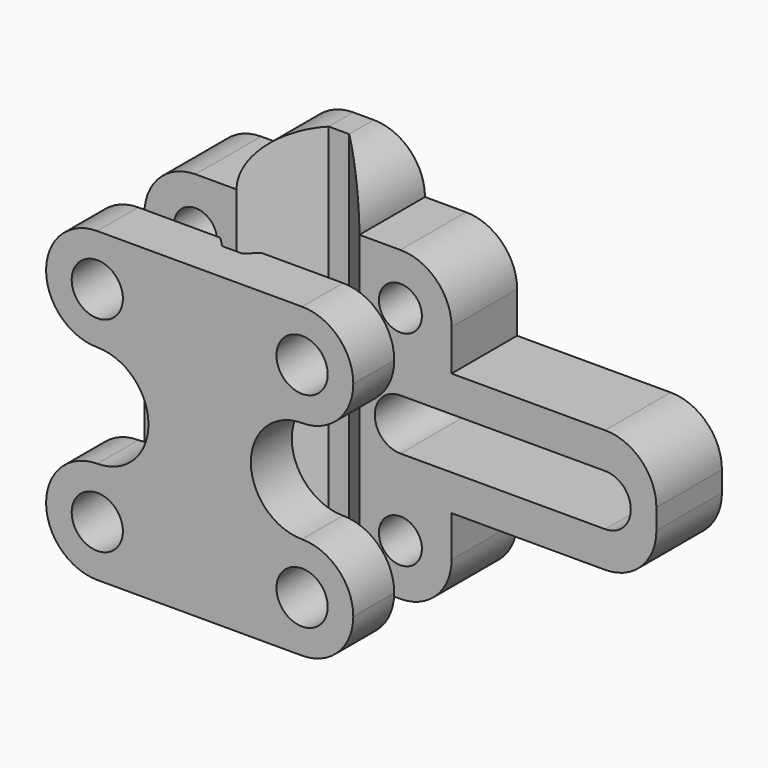
from build123d import *

# Parameters (mm, degrees)
F0_R      = 2.5
F1_DEPTH  = 8
F3_DEPTH  = 40
F4_D      = 4.2
F5_R      = 4.99999
F7_DEPTH  = 5
F8_D      = 5
F9_R      = 5
F11_DEPTH = 50
F13_R     = 4.99999


# Not quite as in the source:
# - a fillet or chamfer is up to 0.001 mm smaller than in the source, because OpenCascade refuses the exact size


with BuildPart() as f1:
    # F0 (on Front) → F1 (new body)
    with BuildSketch(Plane.XZ):
        Polygon((24, 0), (36, 0), (36, 5), (45, 5), (45, 14), (65, 14), (65, 26), (45, 26), (45, 35), (36, 35), (36, 40), (24, 40), (24, 35), (15, 35), (15, 26), (15, 14), (15, 5), (24, 5), align=None)
        with Locations((20, 20)):
            Circle(F0_R, mode=Mode.SUBTRACT)
        with BuildLine():
            ThreePointArc((40, 17.5), (37.5, 20), (40, 22.5))
            Line((40, 22.5), (60, 22.5))
            ThreePointArc((60, 22.5), (62.5, 20), (60, 17.5))
            Line((60, 17.5), (40, 17.5))
        make_face(mode=Mode.SUBTRACT)
    extrude(amount=F1_DEPTH)

    # F2 (on Top) → F3 (cut)
    with BuildSketch(Plane.XY):
        Polygon((29, -3), (24, -8), (36, -8), (31, -3), align=None)
    extrude(amount=F3_DEPTH, mode=Mode.SUBTRACT)

    # F4 (through all)
    with Locations(Plane(origin=(0, 0, 0), x_dir=(1, 0, 0), z_dir=(0, 1, 0))):
        with Locations((20, -30), (40, -30), (40, -10), (20, -10)):
            Hole(F4_D / 2)

    # F5 (radius 5 in the source; OpenCascade refuses exactly that, so slightly less here)
    f5_edges = [f1.edges().sort_by_distance(p)[0] for p in [
        (36, -4, 40),
        (24, -4, 40),
        (45, -4, 35),
        (15, -4, 35),
        (15, -4, 5),
        (36, -4, 0),
        (24, -4, 0),
        (45, -4, 5),
        (65, -4, 26),
        (65, -4, 14),
    ]]
    fillet(f5_edges, radius=F5_R)


with BuildPart() as f7:
    # F6 (on Front) → F7 (new body)
    with BuildSketch(Plane.XZ):
        with BuildLine():
            Line((45, 25), (45, 35))
            Line((45, 35), (15, 35))
            Line((15, 35), (15, 25))
            Line((15, 25), (20, 25))
            ThreePointArc((20, 25), (25, 20), (20, 15))
            Line((20, 15), (15, 15))
            Line((15, 15), (15, 5))
            Line((15, 5), (45, 5))
            Line((45, 5), (45, 15))
            Line((45, 15), (40, 15))
            ThreePointArc((40, 15), (35, 20), (40, 25))
            Line((40, 25), (45, 25))
        make_face()
    extrude(amount=F7_DEPTH)

    # F8 (through all)
    with Locations(Plane(origin=(0, 0, 0), x_dir=(1, 0, 0), z_dir=(0, 1, 0))):
        with Locations((40, -30), (20, -30), (20, -10), (40, -10)):
            Hole(F8_D / 2)

    # F9
    f9_edges = [f7.edges().sort_by_distance(p)[0] for p in [
        (45, -2.5, 35),
        (15, -2.5, 35),
        (45, -2.5, 5),
        (15, -2.5, 5),
    ]]
    fillet(f9_edges, radius=F9_R)

    # F10 (on face) → F11 (cut)
    with BuildSketch(Plane.XY.offset(35)):
        Polygon((32, 0), (28, 0), (29, -1), (31, -1), align=None)
    extrude(amount=-F11_DEPTH, mode=Mode.SUBTRACT)


with BuildPart() as f7_1:
    # F12: moved
    add(f7.part.moved(Location((0, -15, 0))))

    # F13 (radius 5 in the source; OpenCascade refuses exactly that, so slightly less here)
    f13_edges = [f7_1.edges().sort_by_distance(p)[0] for p in [
        (15, -17.5, 25),
        (45, -17.5, 25),
        (45, -17.5, 15),
        (15, -17.5, 15),
    ]]
    fillet(f13_edges, radius=F13_R)


solid = Compound([f1.part, f7_1.part])
